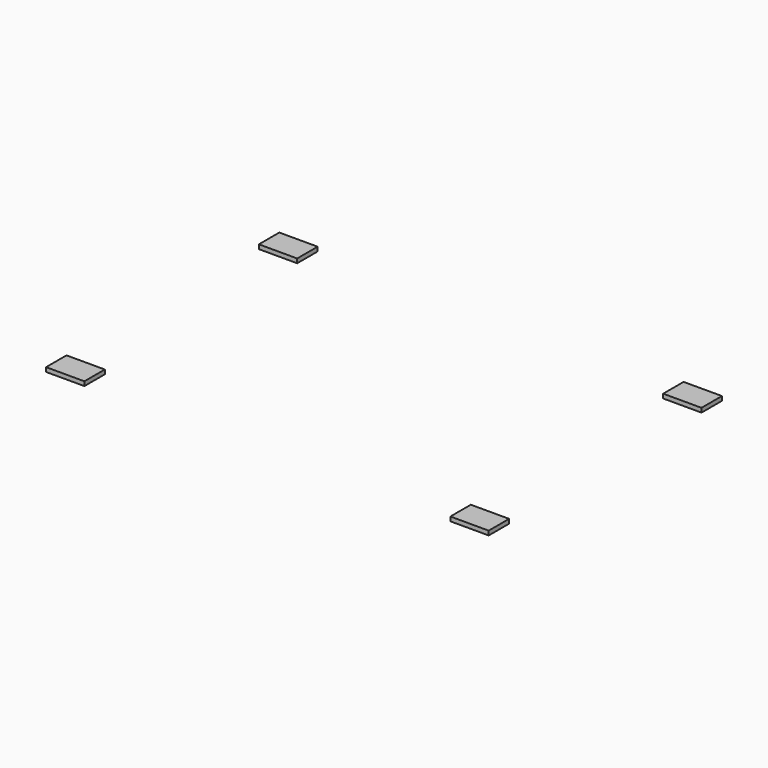
from build123d import *

# Parameters (mm, degrees)
F4_W     = 180
F4_H     = 120
F5_DEPTH = 20


# Not quite as in the source:
# - a feature names something its author has since deleted; it is built from what else it names


with BuildPart() as f5:
    # F4 (on Top) → F5 (new body)
    with BuildSketch(Plane.XY):
        with Locations((-950, -625)):
            Rectangle(F4_W, F4_H)
    extrude(amount=F5_DEPTH)


with BuildPart() as f6_1:
    # F6: instance of F5
    add(f5.part.mirror(Plane.YZ))


with BuildPart() as f7_1:
    # F7: instance of F5
    add(f5.part.mirror(Plane.XZ))


with BuildPart() as f7_2:
    # F7: instance of F6_1
    add(f6_1.part.mirror(Plane.XZ))


solid = Compound([f5.part, f6_1.part, f7_1.part, f7_2.part])
